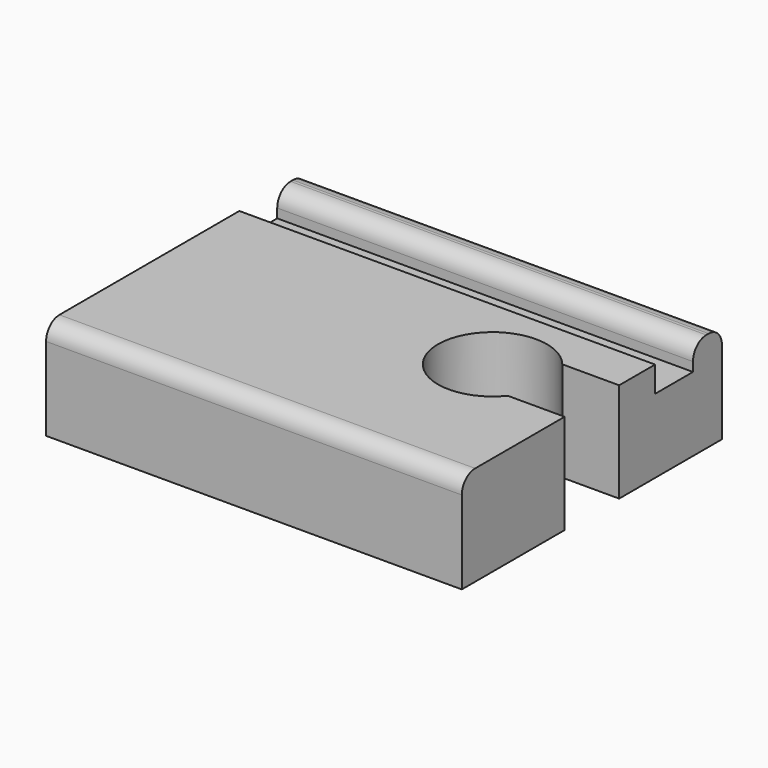
from build123d import *

# Parameters (mm, degrees)
F0_W     = 50
F0_H     = 39.1
F1_DEPTH = 6
F2_W     = 50
F2_H     = 5.7
F3_DEPTH = 3.1
F4_DEPTH = 12
F5_R     = 2


with BuildPart() as f1:
    # F0 (on Top) → F1 (new body, symmetric)
    with BuildSketch(Plane.XY):
        Rectangle(F0_W, F0_H)
    extrude(amount=F1_DEPTH, both=True)

    # F2 (on face) → F3 (cut)
    with BuildSketch(Plane.XY.offset(6)):
        with Locations((0, 12.35)):
            Rectangle(F2_W, F2_H)
    extrude(amount=-F3_DEPTH, mode=Mode.SUBTRACT)

    # F2 (on face) → F4 (cut, through all)
    with BuildSketch(Plane.XY.offset(6)):
        with BuildLine():
            Line((25, -4.1), (25, 0))
            Line((25, 0), (25, 4.1))
            Line((25, 4.1), (18.1580818318, 4.1))
            ThreePointArc((18.1580818318, 4.1), (6.5, 0), (18.1580818318, -4.1))
            Line((18.1580818318, -4.1), (25, -4.1))
        make_face()
    extrude(amount=-F4_DEPTH, mode=Mode.SUBTRACT)

    # F5
    f5_edges = [f1.edges().sort_by_distance(p)[0] for p in [
        (0, -19.55, 6),
        (0, 15.2, 6),
        (0, 19.55, 6),
    ]]
    fillet(f5_edges, radius=F5_R)


solid = f1.part
